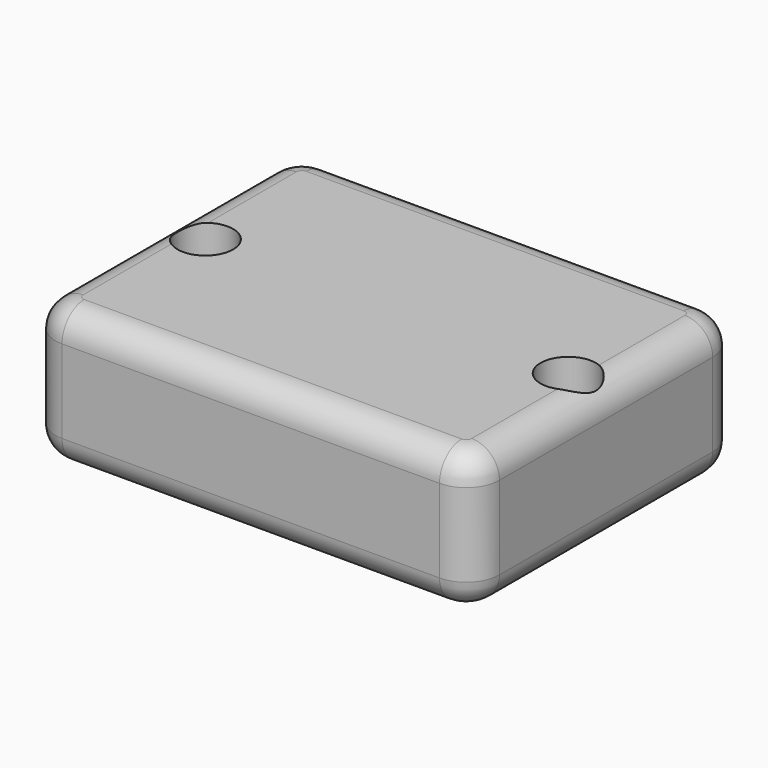
from build123d import *

# Parameters (mm, degrees)
F1_DEPTH     = 25
F2_D         = 10
F3_T1_DEPTH  = 48
F3_T3_DEPTH  = 68
F3_T6_ANGLE  = 90
F3_T8_ANGLE  = 90
F3_T10_ANGLE = 90
F3_T12_ANGLE = 90
F3_T14_ANGLE = 90
F3_T16_ANGLE = 90
F3_T18_ANGLE = 90
F3_T20_ANGLE = 90


# Not quite as in the source:
# - a fillet or chamfer that OpenCascade refuses, or shapes differently, is made with other operations: its cross-section is extruded or revolved along the edge and cut away or added


with BuildPart() as f1:
    # F0 (on Top) → F1 (new body)
    with BuildSketch(Plane.XY):
        with BuildLine():
            ThreePointArc((40, 24), (38.2426406871, 28.2426406871), (34, 30))
            Line((34, 30), (-34, 30))
            ThreePointArc((-34, 30), (-38.2426406871, 28.2426406871), (-40, 24))
            Line((-40, 24), (-40, -24))
            ThreePointArc((-40, -24), (-38.2426406871, -28.2426406871), (-34, -30))
            Line((-34, -30), (34, -30))
            ThreePointArc((34, -30), (38.2426406871, -28.2426406871), (40, -24))
            Line((40, -24), (40, 24))
        make_face()
    extrude(amount=F1_DEPTH)

    # F2 (through all)
    with Locations(Plane(origin=(0, 0, 0), x_dir=(1, 0, 0), z_dir=(0, 0, -1))):
        with Locations((-32.1810245514, 0), (33.1866517663, 0)):
            Hole(F2_D / 2)

    # F3: fillet of radius 5 on 16 edges, made by hand

    # F3_s2 → F3_t1 (cut)
    with BuildSketch(Plane.XZ.offset(-24)):
        with BuildLine():
            ThreePointArc((40, 20), (38.5355339059, 23.5355339059), (35, 25))
            Line((35, 25), (40, 25))
            Line((40, 25), (40, 20))
        make_face()
        with BuildLine():
            ThreePointArc((40, 5), (38.5355339059, 1.4644660941), (35, 0))
            Line((35, 0), (40, 0))
            Line((40, 0), (40, 5))
        make_face()
        with BuildLine():
            ThreePointArc((-35, 0), (-38.5355339059, 1.4644660941), (-40, 5))
            Line((-40, 5), (-40, 0))
            Line((-40, 0), (-35, 0))
        make_face()
        with BuildLine():
            ThreePointArc((-35, 25), (-38.5355339059, 23.5355339059), (-40, 20))
            Line((-40, 20), (-40, 25))
            Line((-40, 25), (-35, 25))
        make_face()
    extrude(amount=F3_T1_DEPTH, mode=Mode.SUBTRACT)

    # F3_s4 → F3_t3 (cut)
    with BuildSketch(Plane.YZ.offset(-34)):
        with BuildLine():
            ThreePointArc((-30, 5), (-28.5355339059, 1.4644660941), (-25, 0))
            Line((-25, 0), (-30, 0))
            Line((-30, 0), (-30, 5))
        make_face()
        with BuildLine():
            ThreePointArc((-30, 20), (-28.5355339059, 23.5355339059), (-25, 25))
            Line((-25, 25), (-30, 25))
            Line((-30, 25), (-30, 20))
        make_face()
        with BuildLine():
            ThreePointArc((25, 0), (28.5355339059, 1.4644660941), (30, 5))
            Line((30, 5), (30, 0))
            Line((30, 0), (25, 0))
        make_face()
        with BuildLine():
            ThreePointArc((25, 25), (28.5355339059, 23.5355339059), (30, 20))
            Line((30, 20), (30, 25))
            Line((30, 25), (25, 25))
        make_face()
    extrude(amount=F3_T3_DEPTH, mode=Mode.SUBTRACT)

    # F3_s5 → F3_t6 (revolve, cut)
    with BuildSketch(Plane.YZ.offset(34)):
        with BuildLine():
            ThreePointArc((-30, 5), (-28.5355339059, 1.4644660941), (-25, 0))
            Line((-25, 0), (-30, 0))
            Line((-30, 0), (-30, 5))
        make_face()
    revolve(axis=Axis((34, -24, 0), (0, 0, 1)), revolution_arc=F3_T6_ANGLE, mode=Mode.SUBTRACT)

    # F3_s7 → F3_t8 (revolve, cut)
    with BuildSketch(Plane.YZ.offset(34)):
        with BuildLine():
            ThreePointArc((-30, 20), (-28.5355339059, 23.5355339059), (-25, 25))
            Line((-25, 25), (-30, 25))
            Line((-30, 25), (-30, 20))
        make_face()
    revolve(axis=Axis((34, -24, 25), (0, 0, 1)), revolution_arc=F3_T8_ANGLE, mode=Mode.SUBTRACT)

    # F3_s9 → F3_t10 (revolve, cut)
    with BuildSketch(Plane.XZ.offset(24)):
        with BuildLine():
            ThreePointArc((-35, 0), (-38.5355339059, 1.4644660941), (-40, 5))
            Line((-40, 5), (-40, 0))
            Line((-40, 0), (-35, 0))
        make_face()
    revolve(axis=Axis((-34, -24, 0), (0, 0, 1)), revolution_arc=F3_T10_ANGLE, mode=Mode.SUBTRACT)

    # F3_s11 → F3_t12 (revolve, cut)
    with BuildSketch(Plane.XZ.offset(-24)):
        with BuildLine():
            ThreePointArc((35, 0), (38.5355339059, 1.4644660941), (40, 5))
            Line((40, 5), (40, 0))
            Line((40, 0), (35, 0))
        make_face()
    revolve(axis=Axis((34, 24, 0), (0, 0, 1)), revolution_arc=F3_T12_ANGLE, mode=Mode.SUBTRACT)

    # F3_s13 → F3_t14 (revolve, cut)
    with BuildSketch(Plane.YZ.offset(-34)):
        with BuildLine():
            ThreePointArc((25, 0), (28.5355339059, 1.4644660941), (30, 5))
            Line((30, 5), (30, 0))
            Line((30, 0), (25, 0))
        make_face()
    revolve(axis=Axis((-34, 24, 0), (0, 0, 1)), revolution_arc=F3_T14_ANGLE, mode=Mode.SUBTRACT)

    # F3_s15 → F3_t16 (revolve, cut)
    with BuildSketch(Plane.XZ.offset(24)):
        with BuildLine():
            ThreePointArc((-35, 25), (-38.5355339059, 23.5355339059), (-40, 20))
            Line((-40, 20), (-40, 25))
            Line((-40, 25), (-35, 25))
        make_face()
    revolve(axis=Axis((-34, -24, 25), (0, 0, 1)), revolution_arc=F3_T16_ANGLE, mode=Mode.SUBTRACT)

    # F3_s17 → F3_t18 (revolve, cut)
    with BuildSketch(Plane.XZ.offset(-24)):
        with BuildLine():
            ThreePointArc((35, 25), (38.5355339059, 23.5355339059), (40, 20))
            Line((40, 20), (40, 25))
            Line((40, 25), (35, 25))
        make_face()
    revolve(axis=Axis((34, 24, 25), (0, 0, 1)), revolution_arc=F3_T18_ANGLE, mode=Mode.SUBTRACT)

    # F3_s19 → F3_t20 (revolve, cut)
    with BuildSketch(Plane.YZ.offset(-34)):
        with BuildLine():
            ThreePointArc((25, 25), (28.5355339059, 23.5355339059), (30, 20))
            Line((30, 20), (30, 25))
            Line((30, 25), (25, 25))
        make_face()
    revolve(axis=Axis((-34, 24, 25), (0, 0, 1)), revolution_arc=F3_T20_ANGLE, mode=Mode.SUBTRACT)


solid = f1.part
